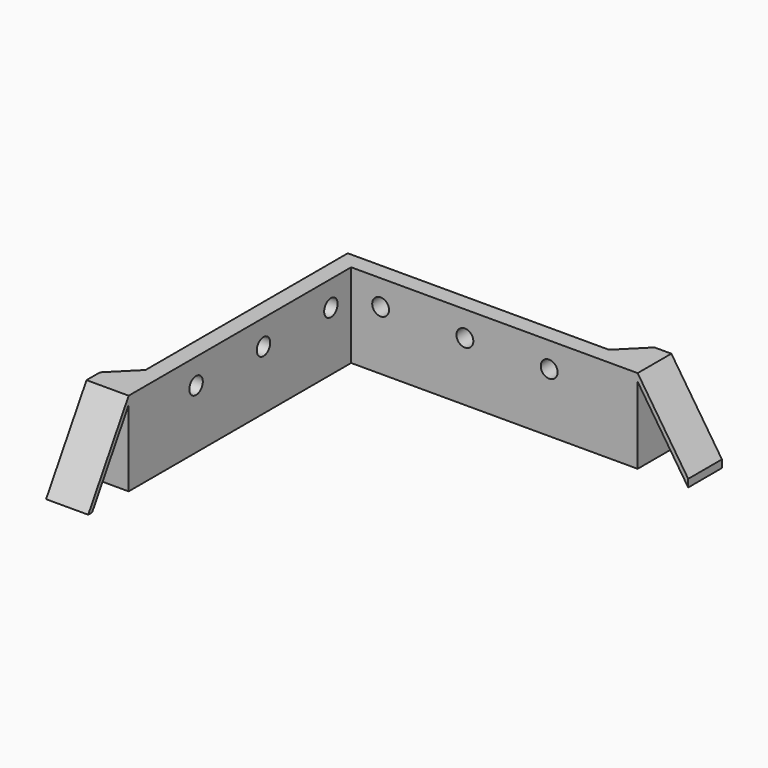
from build123d import *

# Parameters (mm, degrees)
F1_DEPTH  = 10
F2_W      = 2
F2_H      = 10
F3_DEPTH  = 25
F4_DEPTH  = 44.001
F6_DEPTH  = 41.001
F9_DEPTH  = 3
F10_SIZE  = 2.99999
F12_DEPTH = 3
F13_SIZE  = 2.99999
F16_D     = 2
F17_D     = 2


# Not quite as in the source:
# - a fillet or chamfer is up to 0.001 mm smaller than in the source, because OpenCascade refuses the exact size
# - a feature of the source that left no trace in its solid (it failed there, or was rolled back) is left out


with BuildPart() as f1:
    # F0 (on Top) → F1 (new body)
    with BuildSketch(Plane.XY):
        Polygon((-22, -19.5), (-20, -19.5), (-20, 19.5), (20, 19.5), (20, 21.5), (-22, 21.5), align=None)
        Polygon((20, 19.5), (20, -19.5), (-20, -19.5), (-22, -19.5), (-22, -21.5), (22, -21.5), (22, 21.5), (20, 21.5), align=None)
    extrude(amount=-F1_DEPTH)

    # F2 (on face) → F3 (cut)
    with BuildSketch(Plane(origin=(-22, 0, 0), x_dir=(0, -1, 0), z_dir=(-1, 0, 0))):
        with Locations((20.5, -5)):
            Rectangle(F2_W, F2_H)
        Polygon((13.5, -10), (18.9169048105, -10), (13.5, -0.9718253158), align=None)
    extrude(amount=-F3_DEPTH, mode=Mode.SUBTRACT)

    # F2 (on face) → F4 (cut, through all)
    with BuildSketch(Plane(origin=(-22, 0, 0), x_dir=(0, -1, 0), z_dir=(-1, 0, 0))):
        Polygon((19.5, 0), (13.5, 0), (19.5, -10), align=None)
        with Locations((20.5, -5)):
            Rectangle(F2_W, F2_H)
    extrude(amount=-F4_DEPTH, mode=Mode.SUBTRACT)

    # F5 (on face) → F6 (cut, through all)
    with BuildSketch(Plane(origin=(0, 21.5, 0), x_dir=(-1, 0, 0), z_dir=(0, 1, 0))):
        Polygon((-14, -0.9077913453), (-20, -10), (-14, -10), align=None)
        Polygon((-22, -10), (-20, -10), (-20, -9.0922086547), (-14, 0), (-22, 0), align=None)
    extrude(amount=-F6_DEPTH, mode=Mode.SUBTRACT)

    # F8 (on face) → F9 (join)
    with BuildSketch(Plane(origin=(0, 21.5, 0), x_dir=(-1, 0, 0), z_dir=(0, 1, 0))):
        Polygon((-14, -10), (-9, -10), (-9, 0), (-14, 0), (-20, -9.0922086547), (-20, -10), (-14, -0.9077913453), align=None)
    extrude(amount=F9_DEPTH)

    # F10 (size 3 in the source; OpenCascade refuses exactly that, so slightly less here)
    f10_edges = [f1.edges().sort_by_distance(p)[0] for p in [
        (9, 24.5, -5),
    ]]
    chamfer(f10_edges, length=F10_SIZE)

    # F11 (on face) → F12 (join)
    with BuildSketch(Plane(origin=(-22, 0, 0), x_dir=(0, -1, 0), z_dir=(-1, 0, 0))):
        Polygon((13.5, 0), (8.5, 0), (8.5, -10), (13.5, -10), (13.5, -0.9718253158), (18.9169048105, -10), (19.5, -10), align=None)
    extrude(amount=F12_DEPTH)

    # F13 (size 3 in the source; OpenCascade refuses exactly that, so slightly less here)
    f13_edges = [f1.edges().sort_by_distance(p)[0] for p in [
        (-25, -8.5, -5),
    ]]
    chamfer(f13_edges, length=F13_SIZE)

    # F16 (through all)
    with Locations(Plane(origin=(-22, 0, 0), x_dir=(0, -1, 0), z_dir=(-1, 0, 0))):
        with Locations((-6.5, -3), (3.5, -3), (-16.5, -3)):
            Hole(F16_D / 2)

    # F17 (through all)
    with Locations(Plane(origin=(0, 21.5, 0), x_dir=(-1, 0, 0), z_dir=(0, 1, 0))):
        with Locations((-3.5, -3), (6.5, -3), (16.5, -3)):
            Hole(F17_D / 2)


solid = f1.part
